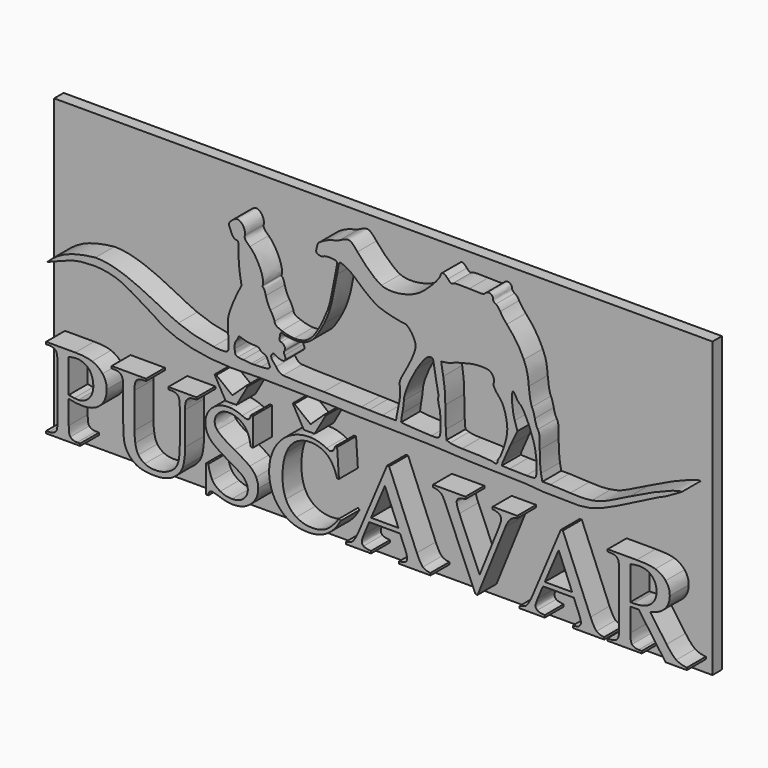
from build123d import *

# Parameters (mm, degrees)
F1_DEPTH = 2
F2_W     = 55.653892
F2_H     = 24.8238056814
F3_DEPTH = 1


# Not quite as in the source:
# - ends of sketch curves that miss each other by under 0.0002 mm in the source are joined


with BuildPart() as f1:
    # F0 (on Front) → F1 (new body)
    with BuildSketch(Plane.XZ):
        with BuildLine():
            add(Edge.make_bspline(
                [(-25.170871, -10.131624), (-25.170873, -10.560896), (-25.124563, -10.827515), (-25.031942, -10.931476)],
                knots=[0, 0, 0, 0, 1, 1, 1, 1], degree=3))
            Line((-25.170871, -10.131624), (-25.170871, -8.14457))
            add(Edge.make_bspline(
                [(-24.565539, -8.250211), (-24.754088, -8.226738), (-24.955865, -8.191524), (-25.170871, -8.14457)],
                knots=[0, 0, 0, 0, 1, 1, 1, 1], degree=3))
            add(Edge.make_bspline(
                [(-24.039596, -8.285425), (-24.201682, -8.285428), (-24.376996, -8.273689), (-24.565539, -8.250211)],
                knots=[0, 0, 0, 0, 1, 1, 1, 1], degree=3))
            add(Edge.make_bspline(
                [(-22.503939, -7.762251), (-22.86615, -8.111038), (-23.378035, -8.285428), (-24.039596, -8.285425)],
                knots=[0, 0, 0, 0, 1, 1, 1, 1], degree=3))
            add(Edge.make_bspline(
                [(-21.96063, -6.40401), (-21.960635, -6.960725), (-22.141738, -7.413473), (-22.503939, -7.762251)],
                knots=[0, 0, 0, 0, 1, 1, 1, 1], degree=3))
            add(Edge.make_bspline(
                [(-22.317874, -5.342571), (-22.079716, -5.641054), (-21.960635, -5.994868), (-21.96063, -6.40401)],
                knots=[0, 0, 0, 0, 1, 1, 1, 1], degree=3))
            add(Edge.make_bspline(
                [(-23.196101, -4.706211), (-22.848784, -4.83198), (-22.556042, -5.0441), (-22.317874, -5.342571)],
                knots=[0, 0, 0, 0, 1, 1, 1, 1], degree=3))
            add(Edge.make_bspline(
                [(-24.620119, -4.517567), (-24.018098, -4.517572), (-23.543426, -4.580454), (-23.196101, -4.706211)],
                knots=[0, 0, 0, 0, 1, 1, 1, 1], degree=3))
            Line((-24.620119, -4.517567), (-27.0861, -4.517567))
            Line((-27.0861, -4.517567), (-27.0861, -4.703696))
            Line((-27.0861, -4.703696), (-26.833052, -4.703696))
            add(Edge.make_bspline(
                [(-26.257491, -4.925038), (-26.386496, -4.777484), (-26.57835, -4.703702), (-26.833052, -4.703696)],
                knots=[0, 0, 0, 0, 1, 1, 1, 1], degree=3))
            add(Edge.make_bspline(
                [(-26.123524, -5.72489), (-26.123525, -5.295626), (-26.16818, -5.029008), (-26.257491, -4.925038)],
                knots=[0, 0, 0, 0, 1, 1, 1, 1], degree=3))
            Line((-26.123524, -5.72489), (-26.123524, -10.131624))
            add(Edge.make_bspline(
                [(-26.222758, -10.87111), (-26.156603, -10.767148), (-26.123525, -10.520652), (-26.123524, -10.131624)],
                knots=[0, 0, 0, 0, 1, 1, 1, 1], degree=3))
            add(Edge.make_bspline(
                [(-26.833052, -11.15282), (-26.548579, -11.15282), (-26.345149, -11.058916), (-26.222758, -10.87111)],
                knots=[0, 0, 0, 0, 1, 1, 1, 1], degree=3))
            Line((-26.833052, -11.15282), (-27.0861, -11.15282))
            Line((-27.0861, -11.15282), (-27.0861, -11.33895))
            Line((-27.0861, -11.33895), (-24.203333, -11.33895))
            Line((-24.203333, -11.33895), (-24.203333, -11.15282))
            Line((-24.203333, -11.15282), (-24.461343, -11.15282))
            add(Edge.make_bspline(
                [(-25.031942, -10.931476), (-24.906248, -11.079038), (-24.716048, -11.15282), (-24.461343, -11.15282)],
                knots=[0, 0, 0, 0, 1, 1, 1, 1], degree=3))
        make_face()
        with BuildLine():
            add(Edge.make_bspline(
                [(-25.170871, -7.857829), (-24.995558, -7.89137), (-24.840091, -7.916522), (-24.704468, -7.933288)],
                knots=[0, 0, 0, 0, 1, 1, 1, 1], degree=3))
            Line((-25.170871, -7.857829), (-25.170871, -5.020616))
            add(Edge.make_bspline(
                [(-24.520884, -4.925035), (-24.689585, -4.925041), (-24.906248, -4.956902), (-25.170871, -5.020616)],
                knots=[0, 0, 0, 0, 1, 1, 1, 1], degree=3))
            add(Edge.make_bspline(
                [(-23.776624, -5.11368), (-23.994943, -4.987922), (-24.24303, -4.925041), (-24.520884, -4.925035)],
                knots=[0, 0, 0, 0, 1, 1, 1, 1], degree=3))
            add(Edge.make_bspline(
                [(-23.270527, -5.682128), (-23.389612, -5.428931), (-23.558311, -5.239448), (-23.776624, -5.11368)],
                knots=[0, 0, 0, 0, 1, 1, 1, 1], degree=3))
            add(Edge.make_bspline(
                [(-23.091905, -6.504618), (-23.091909, -6.2095), (-23.15145, -5.935336), (-23.270527, -5.682128)],
                knots=[0, 0, 0, 0, 1, 1, 1, 1], degree=3))
            add(Edge.make_bspline(
                [(-23.466516, -7.553481), (-23.216779, -7.283515), (-23.091909, -6.933893), (-23.091905, -6.504618)],
                knots=[0, 0, 0, 0, 1, 1, 1, 1], degree=3))
            add(Edge.make_bspline(
                [(-24.357147, -7.958437), (-24.013136, -7.95844), (-23.71626, -7.823456), (-23.466516, -7.553481)],
                knots=[0, 0, 0, 0, 1, 1, 1, 1], degree=3))
            add(Edge.make_bspline(
                [(-24.704468, -7.933288), (-24.56885, -7.950054), (-24.453076, -7.958437), (-24.357147, -7.958437)],
                knots=[0, 0, 0, 0, 1, 1, 1, 1], degree=3))
        make_face(mode=Mode.SUBTRACT)
    extrude(amount=F1_DEPTH)



with BuildPart() as f1b:
    # F0 (on Front) → F1, piece 2 (new body)
    with BuildSketch(Plane.XZ):
        with BuildLine():
            add(Edge.make_bspline(
                [(-14.622226, -4.703696), (-14.886858, -4.703702), (-15.09029, -4.816049), (-15.23252, -5.040741)],
                knots=[0, 0, 0, 0, 1, 1, 1, 1], degree=3))
            Line((-14.622226, -4.703696), (-14.369178, -4.703696))
            Line((-14.369178, -4.703696), (-14.369178, -4.517567))
            Line((-14.369178, -4.517567), (-16.75081, -4.517567))
            Line((-16.75081, -4.517567), (-16.75081, -4.703696))
            Line((-16.75081, -4.703696), (-16.497762, -4.703696))
            add(Edge.make_bspline(
                [(-15.922201, -4.925038), (-16.051211, -4.777484), (-16.243065, -4.703702), (-16.497762, -4.703696)],
                knots=[0, 0, 0, 0, 1, 1, 1, 1], degree=3))
            add(Edge.make_bspline(
                [(-15.783272, -5.72489), (-15.783278, -5.298979), (-15.829587, -5.032364), (-15.922201, -4.925038)],
                knots=[0, 0, 0, 0, 1, 1, 1, 1], degree=3))
            Line((-15.783272, -5.72489), (-15.783272, -8.486644))
            add(Edge.make_bspline(
                [(-15.974299, -10.028498), (-15.846953, -9.724994), (-15.783278, -9.211041), (-15.783272, -8.486644)],
                knots=[0, 0, 0, 0, 1, 1, 1, 1], degree=3))
            add(Edge.make_bspline(
                [(-16.686307, -10.775531), (-16.338991, -10.581019), (-16.101656, -10.332007), (-15.974299, -10.028498)],
                knots=[0, 0, 0, 0, 1, 1, 1, 1], degree=3))
            add(Edge.make_bspline(
                [(-17.8672, -11.067302), (-17.427264, -11.067302), (-17.033633, -10.970044), (-16.686307, -10.775531)],
                knots=[0, 0, 0, 0, 1, 1, 1, 1], degree=3))
            add(Edge.make_bspline(
                [(-18.737984, -10.881172), (-18.501478, -11.005259), (-18.211217, -11.067302), (-17.8672, -11.067302)],
                knots=[0, 0, 0, 0, 1, 1, 1, 1], degree=3))
            add(Edge.make_bspline(
                [(-19.281294, -10.408302), (-19.155599, -10.599464), (-18.974496, -10.757086), (-18.737984, -10.881172)],
                knots=[0, 0, 0, 0, 1, 1, 1, 1], degree=3))
            add(Edge.make_bspline(
                [(-19.541785, -9.608452), (-19.493824, -9.950527), (-19.406993, -10.217145), (-19.281294, -10.408302)],
                knots=[0, 0, 0, 0, 1, 1, 1, 1], degree=3))
            add(Edge.make_bspline(
                [(-19.61373, -8.697926), (-19.613732, -8.962871), (-19.589751, -9.266378), (-19.541785, -9.608452)],
                knots=[0, 0, 0, 0, 1, 1, 1, 1], degree=3))
            Line((-19.61373, -8.697926), (-19.61373, -5.72489))
            add(Edge.make_bspline(
                [(-19.489687, -4.970312), (-19.572384, -5.091051), (-19.613732, -5.342577), (-19.61373, -5.72489)],
                knots=[0, 0, 0, 0, 1, 1, 1, 1], degree=3))
            add(Edge.make_bspline(
                [(-18.894279, -4.703696), (-19.172138, -4.703702), (-19.370607, -4.792574), (-19.489687, -4.970312)],
                knots=[0, 0, 0, 0, 1, 1, 1, 1], degree=3))
            Line((-18.894279, -4.703696), (-18.636269, -4.703696))
            Line((-18.636269, -4.703696), (-18.636269, -4.517567))
            Line((-18.636269, -4.517567), (-21.543844, -4.517567))
            Line((-21.543844, -4.517567), (-21.543844, -4.703696))
            Line((-21.543844, -4.703696), (-21.290796, -4.703696))
            add(Edge.make_bspline(
                [(-20.737563, -4.899886), (-20.851683, -4.769099), (-21.036094, -4.703702), (-21.290796, -4.703696)],
                knots=[0, 0, 0, 0, 1, 1, 1, 1], degree=3))
            add(Edge.make_bspline(
                [(-20.566383, -5.72489), (-20.566384, -5.305686), (-20.623444, -5.030684), (-20.737563, -4.899886)],
                knots=[0, 0, 0, 0, 1, 1, 1, 1], degree=3))
            Line((-20.566383, -5.72489), (-20.566383, -8.391066))
            add(Edge.make_bspline(
                [(-20.407607, -10.071257), (-20.513459, -9.772783), (-20.566384, -9.212717), (-20.566383, -8.391066)],
                knots=[0, 0, 0, 0, 1, 1, 1, 1], degree=3))
            add(Edge.make_bspline(
                [(-19.598845, -11.112576), (-19.979246, -10.854343), (-20.248833, -10.507236), (-20.407607, -10.071257)],
                knots=[0, 0, 0, 0, 1, 1, 1, 1], degree=3))
            add(Edge.make_bspline(
                [(-17.926741, -11.499925), (-18.66108, -11.499925), (-19.218448, -11.370808), (-19.598845, -11.112576)],
                knots=[0, 0, 0, 0, 1, 1, 1, 1], degree=3))
            add(Edge.make_bspline(
                [(-16.326582, -11.094969), (-16.718564, -11.36494), (-17.251949, -11.499925), (-17.926741, -11.499925)],
                knots=[0, 0, 0, 0, 1, 1, 1, 1], degree=3))
            add(Edge.make_bspline(
                [(-15.537666, -10.124079), (-15.671639, -10.501368), (-15.934611, -10.824997), (-16.326582, -11.094969)],
                knots=[0, 0, 0, 0, 1, 1, 1, 1], degree=3))
            add(Edge.make_bspline(
                [(-15.336716, -8.531919), (-15.336722, -9.216074), (-15.403706, -9.746793), (-15.537666, -10.124079)],
                knots=[0, 0, 0, 0, 1, 1, 1, 1], degree=3))
            Line((-15.336716, -8.531919), (-15.336716, -5.765135))
            add(Edge.make_bspline(
                [(-15.23252, -5.040741), (-15.30199, -5.144711), (-15.336722, -5.386175), (-15.336716, -5.765135)],
                knots=[0, 0, 0, 0, 1, 1, 1, 1], degree=3))
        make_face()
    extrude(amount=F1_DEPTH)


with BuildPart() as f1c:
    # F0 (on Front) → F1, piece 3 (new body)
    with BuildSketch(Plane.XZ):
        with BuildLine():
            add(Edge.make_bspline(
                [(-9.779574, -6.720932), (-9.839121, -6.268193), (-9.945798, -5.907672), (-10.099608, -5.639372)],
                knots=[0, 0, 0, 0, 1, 1, 1, 1], degree=3))
            Line((-9.779574, -6.720932), (-9.59599, -6.720932))
            Line((-9.59599, -6.720932), (-9.59599, -4.361619))
            Line((-9.59599, -4.361619), (-9.779574, -4.361619))
            add(Edge.make_bspline(
                [(-9.911059, -4.676027), (-9.856485, -4.624052), (-9.812656, -4.519249), (-9.779574, -4.361619)],
                knots=[0, 0, 0, 0, 1, 1, 1, 1], degree=3))
            add(Edge.make_bspline(
                [(-10.121935, -4.754001), (-10.035935, -4.754006), (-9.965645, -4.728027), (-9.911059, -4.676027)],
                knots=[0, 0, 0, 0, 1, 1, 1, 1], degree=3))
            add(Edge.make_bspline(
                [(-10.51391, -4.628237), (-10.328677, -4.712085), (-10.198019, -4.754006), (-10.121935, -4.754001)],
                knots=[0, 0, 0, 0, 1, 1, 1, 1], degree=3))
            add(Edge.make_bspline(
                [(-11.650148, -4.361619), (-11.292906, -4.361628), (-10.914161, -4.450499), (-10.51391, -4.628237)],
                knots=[0, 0, 0, 0, 1, 1, 1, 1], degree=3))
            add(Edge.make_bspline(
                [(-13.064241, -4.892341), (-12.693768, -4.538533), (-12.222402, -4.361628), (-11.650148, -4.361619)],
                knots=[0, 0, 0, 0, 1, 1, 1, 1], degree=3))
            add(Edge.make_bspline(
                [(-13.619956, -6.157516), (-13.619956, -5.667883), (-13.434718, -5.24616), (-13.064241, -4.892341)],
                knots=[0, 0, 0, 0, 1, 1, 1, 1], degree=3))
            add(Edge.make_bspline(
                [(-13.431411, -6.932214), (-13.557108, -6.697462), (-13.619956, -6.43923), (-13.619956, -6.157516)],
                knots=[0, 0, 0, 0, 1, 1, 1, 1], degree=3))
            add(Edge.make_bspline(
                [(-12.878176, -7.576121), (-13.121302, -7.381611), (-13.305713, -7.166977), (-13.431411, -6.932214)],
                knots=[0, 0, 0, 0, 1, 1, 1, 1], degree=3))
            add(Edge.make_bspline(
                [(-11.650148, -8.358367), (-12.225712, -8.031387), (-12.635053, -7.77064), (-12.878176, -7.576121)],
                knots=[0, 0, 0, 0, 1, 1, 1, 1], degree=3))
            add(Edge.make_bspline(
                [(-10.593298, -8.999759), (-10.722308, -8.899151), (-11.074591, -8.685354), (-11.650148, -8.358367)],
                knots=[0, 0, 0, 0, 1, 1, 1, 1], degree=3))
            add(Edge.make_bspline(
                [(-10.169071, -9.477656), (-10.260041, -9.306622), (-10.401448, -9.147321), (-10.593298, -8.999759)],
                knots=[0, 0, 0, 0, 1, 1, 1, 1], degree=3))
            add(Edge.make_bspline(
                [(-10.032622, -9.985738), (-10.032628, -9.818057), (-10.07811, -9.648697), (-10.169071, -9.477656)],
                knots=[0, 0, 0, 0, 1, 1, 1, 1], degree=3))
            add(Edge.make_bspline(
                [(-10.39235, -10.770501), (-10.152537, -10.549157), (-10.032628, -10.287571), (-10.032622, -9.985738)],
                knots=[0, 0, 0, 0, 1, 1, 1, 1], degree=3))
            add(Edge.make_bspline(
                [(-11.372292, -11.102513), (-10.958816, -11.102516), (-10.632168, -10.991843), (-10.39235, -10.770501)],
                knots=[0, 0, 0, 0, 1, 1, 1, 1], degree=3))
            add(Edge.make_bspline(
                [(-12.357194, -10.86105), (-12.057841, -11.022027), (-11.729539, -11.102516), (-11.372292, -11.102513)],
                knots=[0, 0, 0, 0, 1, 1, 1, 1], degree=3))
            add(Edge.make_bspline(
                [(-13.024547, -10.254872), (-12.879006, -10.498015), (-12.656554, -10.700075), (-12.357194, -10.86105)],
                knots=[0, 0, 0, 0, 1, 1, 1, 1], degree=3))
            add(Edge.make_bspline(
                [(-13.371869, -9.155704), (-13.285866, -9.645343), (-13.170094, -10.011732), (-13.024547, -10.254872)],
                knots=[0, 0, 0, 0, 1, 1, 1, 1], degree=3))
            Line((-13.371869, -9.155704), (-13.555454, -9.155704))
            Line((-13.555454, -9.155704), (-13.555454, -11.494895))
            Line((-13.555454, -11.494895), (-13.371869, -11.494895))
            add(Edge.make_bspline(
                [(-13.265192, -11.183002), (-13.313155, -11.233309), (-13.348715, -11.337273), (-13.371869, -11.494895)],
                knots=[0, 0, 0, 0, 1, 1, 1, 1], degree=3))
            add(Edge.make_bspline(
                [(-13.069202, -11.107546), (-13.151901, -11.107546), (-13.21723, -11.132695), (-13.265192, -11.183002)],
                knots=[0, 0, 0, 0, 1, 1, 1, 1], degree=3))
            add(Edge.make_bspline(
                [(-12.45643, -11.266006), (-12.778944, -11.160365), (-12.983202, -11.107546), (-13.069202, -11.107546)],
                knots=[0, 0, 0, 0, 1, 1, 1, 1], degree=3))
            add(Edge.make_bspline(
                [(-11.818846, -11.449621), (-11.921392, -11.432855), (-12.133919, -11.371647), (-12.45643, -11.266006)],
                knots=[0, 0, 0, 0, 1, 1, 1, 1], degree=3))
            add(Edge.make_bspline(
                [(-11.268095, -11.494895), (-11.463258, -11.494895), (-11.646843, -11.479805), (-11.818846, -11.449621)],
                knots=[0, 0, 0, 0, 1, 1, 1, 1], degree=3))
            add(Edge.make_bspline(
                [(-9.742361, -10.933991), (-10.137651, -11.307927), (-10.646227, -11.494895), (-11.268095, -11.494895)],
                knots=[0, 0, 0, 0, 1, 1, 1, 1], degree=3))
            add(Edge.make_bspline(
                [(-9.149435, -9.59839), (-9.149441, -10.114858), (-9.347082, -10.560058), (-9.742361, -10.933991)],
                knots=[0, 0, 0, 0, 1, 1, 1, 1], degree=3))
            add(Edge.make_bspline(
                [(-9.3355, -8.818659), (-9.211462, -9.066835), (-9.149441, -9.326744), (-9.149435, -9.59839)],
                knots=[0, 0, 0, 0, 1, 1, 1, 1], degree=3))
            add(Edge.make_bspline(
                [(-9.866404, -8.172237), (-9.636516, -8.355016), (-9.459546, -8.570489), (-9.3355, -8.818659)],
                knots=[0, 0, 0, 0, 1, 1, 1, 1], degree=3))
            add(Edge.make_bspline(
                [(-11.153974, -7.384962), (-10.525491, -7.727039), (-10.096303, -7.989466), (-9.866404, -8.172237)],
                knots=[0, 0, 0, 0, 1, 1, 1, 1], degree=3))
            add(Edge.make_bspline(
                [(-12.617687, -6.378858), (-12.412601, -6.630389), (-11.924699, -6.965757), (-11.153974, -7.384962)],
                knots=[0, 0, 0, 0, 1, 1, 1, 1], degree=3))
            add(Edge.make_bspline(
                [(-12.831041, -5.810409), (-12.831041, -6.018343), (-12.759924, -6.207826), (-12.617687, -6.378858)],
                knots=[0, 0, 0, 0, 1, 1, 1, 1], degree=3))
            add(Edge.make_bspline(
                [(-12.493643, -5.0835), (-12.718576, -5.296464), (-12.831041, -5.538766), (-12.831041, -5.810409)],
                knots=[0, 0, 0, 0, 1, 1, 1, 1], degree=3))
            add(Edge.make_bspline(
                [(-11.640225, -4.764063), (-11.98424, -4.764069), (-12.268714, -4.870548), (-12.493643, -5.0835)],
                knots=[0, 0, 0, 0, 1, 1, 1, 1], degree=3))
            add(Edge.make_bspline(
                [(-10.757036, -5.000497), (-11.041512, -4.842881), (-11.335908, -4.764069), (-11.640225, -4.764063)],
                knots=[0, 0, 0, 0, 1, 1, 1, 1], degree=3))
            add(Edge.make_bspline(
                [(-10.099608, -5.639372), (-10.253423, -5.371082), (-10.472568, -5.158124), (-10.757036, -5.000497)],
                knots=[0, 0, 0, 0, 1, 1, 1, 1], degree=3))
        make_face()
    extrude(amount=F1_DEPTH)


with BuildPart() as f1d:
    # F0 (on Front) → F1, piece 4 (new body)
    with BuildSketch(Plane.XZ):
        Polygon((-11.903195, -3.984333), (-10.990236, -3.984333), (-10.052469, -2.319231), (-10.201321, -2.319231), (-11.337559, -3.385699), (-12.692111, -2.319231), (-12.845927, -2.319231), align=None)
    extrude(amount=F1_DEPTH)


with BuildPart() as f1e:
    # F0 (on Front) → F1, piece 5 (new body)
    with BuildSketch(Plane.XZ):
        with BuildLine():
            add(Edge.make_bspline(
                [(-2.480866, -6.680691), (-2.685956, -5.986482), (-2.978698, -5.486786), (-3.359094, -5.181594)],
                knots=[0, 0, 0, 0, 1, 1, 1, 1], degree=3))
            Line((-2.480866, -6.680691), (-2.327053, -6.680691))
            Line((-2.327053, -6.680691), (-2.480866, -4.361619))
            Line((-2.480866, -4.361619), (-2.654528, -4.361619))
            add(Edge.make_bspline(
                [(-2.838113, -4.738908), (-2.752112, -4.648365), (-2.69092, -4.522605), (-2.654528, -4.361619)],
                knots=[0, 0, 0, 0, 1, 1, 1, 1], degree=3))
            add(Edge.make_bspline(
                [(-3.071313, -4.834489), (-2.982006, -4.834495), (-2.904274, -4.802636), (-2.838113, -4.738908)],
                knots=[0, 0, 0, 0, 1, 1, 1, 1], degree=3))
            add(Edge.make_bspline(
                [(-3.369016, -4.723819), (-3.230093, -4.797604), (-3.13086, -4.834495), (-3.071313, -4.834489)],
                knots=[0, 0, 0, 0, 1, 1, 1, 1], degree=3))
            add(Edge.make_bspline(
                [(-4.807918, -4.361619), (-4.321672, -4.361628), (-3.842041, -4.482361), (-3.369016, -4.723819)],
                knots=[0, 0, 0, 0, 1, 1, 1, 1], degree=3))
            add(Edge.make_bspline(
                [(-6.537085, -4.831974), (-6.009488, -4.518411), (-5.433102, -4.361628), (-4.807918, -4.361619)],
                knots=[0, 0, 0, 0, 1, 1, 1, 1], degree=3))
            add(Edge.make_bspline(
                [(-7.779996, -6.157516), (-7.478986, -5.587397), (-7.064681, -5.145549), (-6.537085, -4.831974)],
                knots=[0, 0, 0, 0, 1, 1, 1, 1], degree=3))
            add(Edge.make_bspline(
                [(-8.231515, -8.033899), (-8.231515, -7.353106), (-8.08101, -6.727644), (-7.779996, -6.157516)],
                knots=[0, 0, 0, 0, 1, 1, 1, 1], degree=3))
            add(Edge.make_bspline(
                [(-7.546796, -10.237265), (-8.003275, -9.613482), (-8.231515, -8.879029), (-8.231515, -8.033899)],
                knots=[0, 0, 0, 0, 1, 1, 1, 1], degree=3))
            add(Edge.make_bspline(
                [(-4.95677, -11.494895), (-6.07151, -11.494895), (-6.93485, -11.075685), (-7.546796, -10.237265)],
                knots=[0, 0, 0, 0, 1, 1, 1, 1], degree=3))
            add(Edge.make_bspline(
                [(-3.35413, -11.072332), (-3.804001, -11.35404), (-4.338212, -11.494895), (-4.95677, -11.494895)],
                knots=[0, 0, 0, 0, 1, 1, 1, 1], degree=3))
            add(Edge.make_bspline(
                [(-2.17324, -9.739245), (-2.510643, -10.346261), (-2.904274, -10.790624), (-3.35413, -11.072332)],
                knots=[0, 0, 0, 0, 1, 1, 1, 1], degree=3))
            Line((-2.17324, -9.739245), (-2.327053, -9.638634))
            add(Edge.make_bspline(
                [(-3.428558, -10.767986), (-3.094473, -10.578504), (-2.727304, -10.202053), (-2.327053, -9.638634)],
                knots=[0, 0, 0, 0, 1, 1, 1, 1], degree=3))
            add(Edge.make_bspline(
                [(-4.584642, -11.052209), (-4.148013, -11.052209), (-3.762653, -10.957469), (-3.428558, -10.767986)],
                knots=[0, 0, 0, 0, 1, 1, 1, 1], degree=3))
            add(Edge.make_bspline(
                [(-5.92679, -10.690013), (-5.534815, -10.931476), (-5.087434, -11.052209), (-4.584642, -11.052209)],
                knots=[0, 0, 0, 0, 1, 1, 1, 1], degree=3))
            add(Edge.make_bspline(
                [(-6.807499, -9.648694), (-6.612339, -10.101442), (-6.31877, -10.448549), (-5.92679, -10.690013)],
                knots=[0, 0, 0, 0, 1, 1, 1, 1], degree=3))
            add(Edge.make_bspline(
                [(-7.100241, -8.043959), (-7.100241, -8.661038), (-7.002662, -9.195951), (-6.807499, -9.648694)],
                knots=[0, 0, 0, 0, 1, 1, 1, 1], degree=3))
            add(Edge.make_bspline(
                [(-6.790132, -6.167576), (-6.996871, -6.670634), (-7.100241, -7.296093), (-7.100241, -8.043959)],
                knots=[0, 0, 0, 0, 1, 1, 1, 1], degree=3))
            add(Edge.make_bspline(
                [(-5.939195, -5.068408), (-6.29975, -5.298141), (-6.583393, -5.664529), (-6.790132, -6.167576)],
                knots=[0, 0, 0, 0, 1, 1, 1, 1], degree=3))
            add(Edge.make_bspline(
                [(-4.728533, -4.723819), (-5.17509, -4.723824), (-5.578643, -4.838687), (-5.939195, -5.068408)],
                knots=[0, 0, 0, 0, 1, 1, 1, 1], degree=3))
            add(Edge.make_bspline(
                [(-3.359094, -5.181594), (-3.739499, -4.876416), (-4.195975, -4.723824), (-4.728533, -4.723819)],
                knots=[0, 0, 0, 0, 1, 1, 1, 1], degree=3))
        make_face()
    extrude(amount=F1_DEPTH)


with BuildPart() as f1f:
    # F0 (on Front) → F1, piece 6 (new body)
    with BuildSketch(Plane.XZ):
        Polygon((-5.29417, -3.984333), (-4.381211, -3.984333), (-3.443444, -2.319231), (-3.592295, -2.319231), (-4.728533, -3.385699), (-6.083086, -2.319231), (-6.236898, -2.319231), align=None)
    extrude(amount=F1_DEPTH)


with BuildPart() as f1g:
    # F0 (on Front) → F1, piece 7 (new body)
    with BuildSketch(Plane.XZ):
        with BuildLine():
            add(Edge.make_bspline(
                [(-0.223279, -10.131624), (-0.335746, -10.396565), (-0.391977, -10.594434), (-0.391977, -10.725227)],
                knots=[0, 0, 0, 0, 1, 1, 1, 1], degree=3))
            Line((-0.223279, -10.131624), (0.233201, -9.055093))
            Line((0.233201, -9.055093), (2.838112, -9.055093))
            Line((2.838112, -9.055093), (3.244973, -10.036045))
            add(Edge.make_bspline(
                [(3.443444, -10.735287), (3.443438, -10.587725), (3.377282, -10.354644), (3.244973, -10.036045)],
                knots=[0, 0, 0, 0, 1, 1, 1, 1], degree=3))
            add(Edge.make_bspline(
                [(3.302034, -11.016995), (3.396302, -10.939862), (3.443438, -10.845958), (3.443444, -10.735287)],
                knots=[0, 0, 0, 0, 1, 1, 1, 1], degree=3))
            add(Edge.make_bspline(
                [(2.758724, -11.15282), (3.026652, -11.139407), (3.207757, -11.09413), (3.302034, -11.016995)],
                knots=[0, 0, 0, 0, 1, 1, 1, 1], degree=3))
            Line((2.758724, -11.15282), (2.758724, -11.33895))
            Line((2.758724, -11.33895), (5.413249, -11.33895))
            Line((5.413249, -11.33895), (5.413249, -11.15282))
            add(Edge.make_bspline(
                [(4.770707, -10.923931), (4.924514, -11.059754), (5.138695, -11.136051), (5.413249, -11.15282)],
                knots=[0, 0, 0, 0, 1, 1, 1, 1], degree=3))
            add(Edge.make_bspline(
                [(4.257167, -10.036045), (4.445707, -10.492147), (4.616886, -10.788109), (4.770707, -10.923931)],
                knots=[0, 0, 0, 0, 1, 1, 1, 1], degree=3))
            Line((4.257167, -10.036045), (1.915228, -4.361619))
            Line((1.915228, -4.361619), (1.741569, -4.361619))
            Line((1.741569, -4.361619), (-0.625178, -9.975679))
            add(Edge.make_bspline(
                [(-1.185854, -10.956628), (-1.017155, -10.795653), (-0.830264, -10.468671), (-0.625178, -9.975679)],
                knots=[0, 0, 0, 0, 1, 1, 1, 1], degree=3))
            add(Edge.make_bspline(
                [(-1.731644, -11.15282), (-1.450481, -11.102516), (-1.26855, -11.037117), (-1.185854, -10.956628)],
                knots=[0, 0, 0, 0, 1, 1, 1, 1], degree=3))
            Line((-1.731644, -11.15282), (-1.731644, -11.33895))
            Line((-1.731644, -11.33895), (0.387016, -11.33895))
            Line((0.387016, -11.33895), (0.387016, -11.15282))
            add(Edge.make_bspline(
                [(-0.245606, -10.99939), (-0.148028, -11.0782), (0.062846, -11.129345), (0.387016, -11.15282)],
                knots=[0, 0, 0, 0, 1, 1, 1, 1], degree=3))
            add(Edge.make_bspline(
                [(-0.391977, -10.725227), (-0.391977, -10.829191), (-0.343188, -10.920578), (-0.245606, -10.99939)],
                knots=[0, 0, 0, 0, 1, 1, 1, 1], degree=3))
        make_face()
        Polygon((1.557984, -5.926112), (2.699183, -8.682837), (0.387016, -8.682837), align=None, mode=Mode.SUBTRACT)
    extrude(amount=F1_DEPTH)


with BuildPart() as f1h:
    # F0 (on Front) → F1, piece 8 (new body)
    with BuildSketch(Plane.XZ):
        with BuildLine():
            add(Edge.make_bspline(
                [(12.746691, -4.703696), (12.508521, -4.7473), (12.328246, -4.824435), (12.205862, -4.9351)],
                knots=[0, 0, 0, 0, 1, 1, 1, 1], degree=3))
            Line((12.746691, -4.703696), (12.746691, -4.517567))
            Line((12.746691, -4.517567), (10.672686, -4.517567))
            Line((10.672686, -4.517567), (10.672686, -4.703696))
            add(Edge.make_bspline(
                [(10.757035, -4.718786), (10.740499, -4.715433), (10.712375, -4.710403), (10.672686, -4.703696)],
                knots=[0, 0, 0, 0, 1, 1, 1, 1], degree=3))
            add(Edge.make_bspline(
                [(11.243287, -4.907431), (11.147353, -4.818564), (10.98527, -4.755683), (10.757035, -4.718786)],
                knots=[0, 0, 0, 0, 1, 1, 1, 1], degree=3))
            add(Edge.make_bspline(
                [(11.387177, -5.186626), (11.387172, -5.089374), (11.339206, -4.996311), (11.243287, -4.907431)],
                knots=[0, 0, 0, 0, 1, 1, 1, 1], degree=3))
            add(Edge.make_bspline(
                [(11.153974, -5.996539), (11.309437, -5.607519), (11.387172, -5.337547), (11.387177, -5.186626)],
                knots=[0, 0, 0, 0, 1, 1, 1, 1], degree=3))
            Line((11.153974, -5.996539), (9.56622, -9.945497))
            Line((9.56622, -9.945497), (7.854423, -5.946234))
            add(Edge.make_bspline(
                [(7.626184, -5.161472), (7.626181, -5.329164), (7.702262, -5.59075), (7.854423, -5.946234)],
                knots=[0, 0, 0, 0, 1, 1, 1, 1], degree=3))
            add(Edge.make_bspline(
                [(7.76511, -4.864671), (7.67249, -4.941812), (7.626181, -5.040747), (7.626184, -5.161472)],
                knots=[0, 0, 0, 0, 1, 1, 1, 1], degree=3))
            add(Edge.make_bspline(
                [(8.370444, -4.703696), (8.059506, -4.733884), (7.857728, -4.787544), (7.76511, -4.864671)],
                knots=[0, 0, 0, 0, 1, 1, 1, 1], degree=3))
            Line((8.370444, -4.703696), (8.370444, -4.517567))
            Line((8.370444, -4.517567), (5.621642, -4.517567))
            Line((5.621642, -4.517567), (5.621642, -4.703696))
            add(Edge.make_bspline(
                [(6.110374, -4.816882), (5.989638, -4.758201), (5.826727, -4.720471), (5.621642, -4.703696)],
                knots=[0, 0, 0, 0, 1, 1, 1, 1], degree=3))
            add(Edge.make_bspline(
                [(6.415519, -5.060863), (6.332823, -4.956905), (6.231107, -4.875578), (6.110374, -4.816882)],
                knots=[0, 0, 0, 0, 1, 1, 1, 1], degree=3))
            add(Edge.make_bspline(
                [(6.688417, -5.61422), (6.559409, -5.312395), (6.468445, -5.127942), (6.415519, -5.060863)],
                knots=[0, 0, 0, 0, 1, 1, 1, 1], degree=3))
            Line((6.688417, -5.61422), (9.208976, -11.494895))
            Line((9.208976, -11.494895), (9.392561, -11.494895))
            Line((9.392561, -11.494895), (11.739461, -5.689679))
            add(Edge.make_bspline(
                [(12.205862, -4.9351), (12.030541, -5.099437), (11.875074, -5.350963), (11.739461, -5.689679)],
                knots=[0, 0, 0, 0, 1, 1, 1, 1], degree=3))
        make_face()
    extrude(amount=F1_DEPTH)


with BuildPart() as f1i:
    # F0 (on Front) → F1, piece 9 (new body)
    with BuildSketch(Plane.XZ):
        with BuildLine():
            add(Edge.make_bspline(
                [(14.463452, -10.131624), (14.350984, -10.396565), (14.294753, -10.594434), (14.294753, -10.725227)],
                knots=[0, 0, 0, 0, 1, 1, 1, 1], degree=3))
            Line((14.463452, -10.131624), (14.919931, -9.055093))
            Line((14.919931, -9.055093), (17.524843, -9.055093))
            Line((17.524843, -9.055093), (17.931704, -10.036045))
            add(Edge.make_bspline(
                [(18.130174, -10.735287), (18.130169, -10.587725), (18.064013, -10.354644), (17.931704, -10.036045)],
                knots=[0, 0, 0, 0, 1, 1, 1, 1], degree=3))
            add(Edge.make_bspline(
                [(17.988764, -11.016995), (18.083033, -10.939862), (18.130169, -10.845958), (18.130174, -10.735287)],
                knots=[0, 0, 0, 0, 1, 1, 1, 1], degree=3))
            add(Edge.make_bspline(
                [(17.445455, -11.15282), (17.713383, -11.139407), (17.894487, -11.09413), (17.988764, -11.016995)],
                knots=[0, 0, 0, 0, 1, 1, 1, 1], degree=3))
            Line((17.445455, -11.15282), (17.445455, -11.33895))
            Line((17.445455, -11.33895), (20.099983, -11.33895))
            Line((20.099983, -11.33895), (20.099983, -11.15282))
            add(Edge.make_bspline(
                [(19.457438, -10.923931), (19.611245, -11.059754), (19.825426, -11.136051), (20.099983, -11.15282)],
                knots=[0, 0, 0, 0, 1, 1, 1, 1], degree=3))
            add(Edge.make_bspline(
                [(18.943898, -10.036045), (19.132438, -10.492147), (19.303617, -10.788109), (19.457438, -10.923931)],
                knots=[0, 0, 0, 0, 1, 1, 1, 1], degree=3))
            Line((18.943898, -10.036045), (16.601959, -4.361619))
            Line((16.601959, -4.361619), (16.428299, -4.361619))
            Line((16.428299, -4.361619), (14.061552, -9.975679))
            add(Edge.make_bspline(
                [(13.500877, -10.956628), (13.669575, -10.795653), (13.856467, -10.468671), (14.061552, -9.975679)],
                knots=[0, 0, 0, 0, 1, 1, 1, 1], degree=3))
            add(Edge.make_bspline(
                [(12.955087, -11.15282), (13.23625, -11.102516), (13.418181, -11.037117), (13.500877, -10.956628)],
                knots=[0, 0, 0, 0, 1, 1, 1, 1], degree=3))
            Line((12.955087, -11.15282), (12.955087, -11.33895))
            Line((12.955087, -11.33895), (15.073747, -11.33895))
            Line((15.073747, -11.33895), (15.073747, -11.15282))
            add(Edge.make_bspline(
                [(14.441124, -10.99939), (14.538703, -11.0782), (14.749576, -11.129345), (15.073747, -11.15282)],
                knots=[0, 0, 0, 0, 1, 1, 1, 1], degree=3))
            add(Edge.make_bspline(
                [(14.294753, -10.725227), (14.294753, -10.829191), (14.343543, -10.920578), (14.441124, -10.99939)],
                knots=[0, 0, 0, 0, 1, 1, 1, 1], degree=3))
        make_face()
        Polygon((16.244715, -5.926112), (17.385914, -8.682837), (15.073747, -8.682837), align=None, mode=Mode.SUBTRACT)
    extrude(amount=F1_DEPTH)


with BuildPart() as f1j:
    # F0 (on Front) → F1, piece 10 (new body)
    with BuildSketch(Plane.XZ):
        with BuildLine():
            add(Edge.make_bspline(
                [(23.012517, -8.1496), (22.843815, -8.156306), (22.70654, -8.159659), (22.600692, -8.159659)],
                knots=[0, 0, 0, 0, 1, 1, 1, 1], degree=3))
            Line((23.012517, -8.1496), (25.289951, -11.33895))
            Line((25.289951, -11.33895), (27.0861, -11.33895))
            Line((27.0861, -11.33895), (27.0861, -11.152764))
            add(Edge.make_bspline(
                [(26.192988, -10.871053), (26.421222, -11.018617), (26.718925, -11.112519), (27.0861, -11.152764)],
                knots=[0, 0, 0, 0, 1, 1, 1, 1], degree=3))
            add(Edge.make_bspline(
                [(25.3743, -9.975622), (25.691847, -10.425017), (25.964742, -10.723494), (26.192988, -10.871053)],
                knots=[0, 0, 0, 0, 1, 1, 1, 1], degree=3))
            Line((25.3743, -9.975622), (23.985017, -8.01875))
            add(Edge.make_bspline(
                [(25.237854, -7.364783), (24.968261, -7.673325), (24.550648, -7.891313), (23.985017, -8.01875)],
                knots=[0, 0, 0, 0, 1, 1, 1, 1], degree=3))
            add(Edge.make_bspline(
                [(25.642234, -6.27316), (25.642228, -6.692376), (25.507436, -7.056249), (25.237854, -7.364783)],
                knots=[0, 0, 0, 0, 1, 1, 1, 1], degree=3))
            add(Edge.make_bspline(
                [(25.28747, -5.259511), (25.523976, -5.542904), (25.642228, -5.880787), (25.642234, -6.27316)],
                knots=[0, 0, 0, 0, 1, 1, 1, 1], degree=3))
            add(Edge.make_bspline(
                [(24.42413, -4.67597), (24.763175, -4.781619), (25.050956, -4.976132), (25.28747, -5.259511)],
                knots=[0, 0, 0, 0, 1, 1, 1, 1], degree=3))
            add(Edge.make_bspline(
                [(22.843818, -4.51751), (23.558304, -4.517516), (24.085074, -4.570337), (24.42413, -4.67597)],
                knots=[0, 0, 0, 0, 1, 1, 1, 1], degree=3))
            Line((22.843818, -4.51751), (20.392722, -4.51751))
            Line((20.392722, -4.51751), (20.392722, -4.70364))
            Line((20.392722, -4.70364), (20.64577, -4.70364))
            add(Edge.make_bspline(
                [(21.221332, -4.924981), (21.092324, -4.777428), (20.900471, -4.703645), (20.64577, -4.70364)],
                knots=[0, 0, 0, 0, 1, 1, 1, 1], degree=3))
            add(Edge.make_bspline(
                [(21.360258, -5.724833), (21.360258, -5.295569), (21.313949, -5.028951), (21.221332, -4.924981)],
                knots=[0, 0, 0, 0, 1, 1, 1, 1], degree=3))
            Line((21.360258, -5.724833), (21.360258, -10.131567))
            add(Edge.make_bspline(
                [(21.256062, -10.871053), (21.325525, -10.767091), (21.360258, -10.520595), (21.360258, -10.131567)],
                knots=[0, 0, 0, 0, 1, 1, 1, 1], degree=3))
            add(Edge.make_bspline(
                [(20.64577, -11.152764), (20.930241, -11.152764), (21.133672, -11.058859), (21.256062, -10.871053)],
                knots=[0, 0, 0, 0, 1, 1, 1, 1], degree=3))
            Line((20.64577, -11.152764), (20.392722, -11.152764))
            Line((20.392722, -11.152764), (20.392722, -11.338893))
            Line((20.392722, -11.338893), (23.275487, -11.338893))
            Line((23.275487, -11.338893), (23.275487, -11.152764))
            Line((23.275487, -11.152764), (23.012517, -11.152764))
            add(Edge.make_bspline(
                [(22.446877, -10.931419), (22.572574, -11.078981), (22.76112, -11.152764), (23.012517, -11.152764)],
                knots=[0, 0, 0, 0, 1, 1, 1, 1], degree=3))
            add(Edge.make_bspline(
                [(22.30795, -10.131567), (22.307948, -10.560839), (22.354257, -10.827458), (22.446877, -10.931419)],
                knots=[0, 0, 0, 0, 1, 1, 1, 1], degree=3))
            Line((22.30795, -10.131567), (22.30795, -8.149543))
            add(Edge.make_bspline(
                [(22.461763, -8.157102), (22.412144, -8.155397), (22.360874, -8.152925), (22.30795, -8.149543)],
                knots=[0, 0, 0, 0, 1, 1, 1, 1], degree=3))
            add(Edge.make_bspline(
                [(22.600692, -8.159659), (22.557688, -8.159662), (22.511379, -8.158807), (22.461763, -8.157102)],
                knots=[0, 0, 0, 0, 1, 1, 1, 1], degree=3))
        make_face()
        with BuildLine():
            add(Edge.make_bspline(
                [(22.30795, -7.832677), (22.370796, -7.83268), (22.425376, -7.83353), (22.471688, -7.835235)],
                knots=[0, 0, 0, 0, 1, 1, 1, 1], degree=3))
            Line((22.30795, -7.832677), (22.30795, -4.995552))
            add(Edge.make_bspline(
                [(23.086941, -4.899971), (22.895085, -4.899977), (22.635423, -4.931838), (22.30795, -4.995552)],
                knots=[0, 0, 0, 0, 1, 1, 1, 1], degree=3))
            add(Edge.make_bspline(
                [(24.131388, -5.299897), (23.868412, -5.033287), (23.520263, -4.899977), (23.086941, -4.899971)],
                knots=[0, 0, 0, 0, 1, 1, 1, 1], degree=3))
            add(Edge.make_bspline(
                [(24.525846, -6.338698), (24.52584, -5.912787), (24.394355, -5.566521), (24.131388, -5.299897)],
                knots=[0, 0, 0, 0, 1, 1, 1, 1], degree=3))
            add(Edge.make_bspline(
                [(24.037114, -7.415229), (24.36293, -7.133527), (24.52584, -6.774683), (24.525846, -6.338698)],
                knots=[0, 0, 0, 0, 1, 1, 1, 1], degree=3))
            add(Edge.make_bspline(
                [(22.585806, -7.837792), (23.227521, -7.837798), (23.71129, -7.696943), (24.037114, -7.415229)],
                knots=[0, 0, 0, 0, 1, 1, 1, 1], degree=3))
            add(Edge.make_bspline(
                [(22.471688, -7.835235), (22.517994, -7.83694), (22.556034, -7.837792), (22.585806, -7.837792)],
                knots=[0, 0, 0, 0, 1, 1, 1, 1], degree=3))
        make_face(mode=Mode.SUBTRACT)
    extrude(amount=F1_DEPTH)


with BuildPart() as f1k:
    # F0 (on Front) → F1, piece 11 (new body)
    with BuildSketch(Plane.XZ):
        with BuildLine():
            add(Edge.make_bspline(
                [(14.899742, -2.01623), (14.315567, -1.917706), (13.141794, -1.861118), (11.129629, -1.83447)],
                knots=[0, 0, 0, 0, 1, 1, 1, 1], degree=3))
            add(Edge.make_bspline(
                [(17.925147, -2.055885), (17.114303, -2.060683), (15.465705, -2.05295), (14.899742, -2.01623)],
                knots=[0, 0, 0, 0, 1, 1, 1, 1], degree=3))
            add(Edge.make_bspline(
                [(21.214684, -1.01897), (18.988603, -2.129127), (18.695713, -1.927172), (17.925147, -2.055885)],
                knots=[0, 0, 0, 0, 1, 1, 1, 1], degree=3))
            add(Edge.make_bspline(
                [(24.843422, 0.821794), (24.0324, 0.446125), (23.120621, -0.068468), (21.214684, -1.01897)],
                knots=[0, 0, 0, 0, 1, 1, 1, 1], degree=3))
            add(Edge.make_bspline(
                [(26.64895, 1.778186), (25.573248, 1.153286), (25.163936, 0.91725), (24.843422, 0.821794)],
                knots=[0, 0, 0, 0, 1, 1, 1, 1], degree=3))
            add(Edge.make_bspline(
                [(22.260445, 0.01807), (24.459105, 1.134149), (26.329982, 1.88451), (26.64895, 1.778186)],
                knots=[0, 0, 0, 0, 1, 1, 1, 1], degree=3))
            add(Edge.make_bspline(
                [(19.075084, -1.308662), (19.829797, -1.192646), (20.08362, -1.086926), (22.260445, 0.01807)],
                knots=[0, 0, 0, 0, 1, 1, 1, 1], degree=3))
            add(Edge.make_bspline(
                [(17.237152, -1.361023), (17.953776, -1.412909), (18.497725, -1.397413), (19.075084, -1.308662)],
                knots=[0, 0, 0, 0, 1, 1, 1, 1], degree=3))
            add(Edge.make_bspline(
                [(15.54574, -1.286872), (15.916188, -1.287134), (16.677324, -1.32049), (17.237152, -1.361023)],
                knots=[0, 0, 0, 0, 1, 1, 1, 1], degree=3))
            Line((15.54574, -1.286872), (14.8722, -1.286307))
            Line((14.8722, -1.286307), (14.753269, -0.709789))
            add(Edge.make_bspline(
                [(14.646597, 1.023368), (14.639852, 0.387217), (14.687858, -0.392704), (14.753269, -0.709789)],
                knots=[0, 0, 0, 0, 1, 1, 1, 1], degree=3))
            add(Edge.make_bspline(
                [(14.475681, 2.481218), (14.632946, 2.222612), (14.657121, 2.016407), (14.646597, 1.023368)],
                knots=[0, 0, 0, 0, 1, 1, 1, 1], degree=3))
            add(Edge.make_bspline(
                [(14.230288, 3.209637), (14.264508, 2.97467), (14.374933, 2.646883), (14.475681, 2.481218)],
                knots=[0, 0, 0, 0, 1, 1, 1, 1], degree=3))
            add(Edge.make_bspline(
                [(13.992815, 3.98485), (14.089208, 3.793447), (14.196072, 3.444601), (14.230288, 3.209637)],
                knots=[0, 0, 0, 0, 1, 1, 1, 1], degree=3))
            add(Edge.make_bspline(
                [(13.720931, 5.435077), (13.784231, 4.713), (13.878002, 4.212832), (13.992815, 3.98485)],
                knots=[0, 0, 0, 0, 1, 1, 1, 1], degree=3))
            add(Edge.make_bspline(
                [(13.301921, 7.281228), (13.569888, 6.662874), (13.640616, 6.351252), (13.720931, 5.435077)],
                knots=[0, 0, 0, 0, 1, 1, 1, 1], degree=3))
            add(Edge.make_bspline(
                [(11.86644, 9.452045), (12.519251, 8.738833), (12.957396, 8.076243), (13.301921, 7.281228)],
                knots=[0, 0, 0, 0, 1, 1, 1, 1], degree=3))
            add(Edge.make_bspline(
                [(11.305868, 10.220463), (11.391271, 10.041367), (11.64353, 9.69558), (11.86644, 9.452045)],
                knots=[0, 0, 0, 0, 1, 1, 1, 1], degree=3))
            add(Edge.make_bspline(
                [(10.928037, 10.647493), (11.05044, 10.591723), (11.220462, 10.399561), (11.305868, 10.220463)],
                knots=[0, 0, 0, 0, 1, 1, 1, 1], degree=3))
            add(Edge.make_bspline(
                [(10.705491, 10.920569), (10.705491, 10.826145), (10.805637, 10.703263), (10.928037, 10.647493)],
                knots=[0, 0, 0, 0, 1, 1, 1, 1], degree=3))
            add(Edge.make_bspline(
                [(10.034742, 11.163841), (10.272082, 11.44982), (10.705491, 11.292625), (10.705491, 10.920569)],
                knots=[0, 0, 0, 0, 1, 1, 1, 1], degree=3))
            add(Edge.make_bspline(
                [(8.692208, 11.063235), (9.745532, 11.016389), (9.923431, 11.029718), (10.034742, 11.163841)],
                knots=[0, 0, 0, 0, 1, 1, 1, 1], degree=3))
            add(Edge.make_bspline(
                [(7.309452, 11.011983), (7.423238, 11.083044), (7.872434, 11.099692), (8.692208, 11.063235)],
                knots=[0, 0, 0, 0, 1, 1, 1, 1], degree=3))
            add(Edge.make_bspline(
                [(6.88839, 11.206843), (7.098428, 10.957226), (7.169275, 10.924441), (7.309452, 11.011983)],
                knots=[0, 0, 0, 0, 1, 1, 1, 1], degree=3))
            add(Edge.make_bspline(
                [(6.246961, 11.24776), (6.317624, 11.598559), (6.572462, 11.582303), (6.88839, 11.206843)],
                knots=[0, 0, 0, 0, 1, 1, 1, 1], degree=3))
            add(Edge.make_bspline(
                [(4.472156, 9.394534), (5.15707, 9.8464), (6.179795, 10.914315), (6.246961, 11.24776)],
                knots=[0, 0, 0, 0, 1, 1, 1, 1], degree=3))
            add(Edge.make_bspline(
                [(1.265395, 8.899809), (2.045132, 8.556449), (3.554869, 8.789365), (4.472156, 9.394534)],
                knots=[0, 0, 0, 0, 1, 1, 1, 1], degree=3))
            add(Edge.make_bspline(
                [(-0.759002, 10.729902), (-0.098001, 9.912098), (0.790384, 9.108981), (1.265395, 8.899809)],
                knots=[0, 0, 0, 0, 1, 1, 1, 1], degree=3))
            add(Edge.make_bspline(
                [(-2.232341, 11.127844), (-1.480111, 11.519927), (-1.374492, 11.4914), (-0.759002, 10.729902)],
                knots=[0, 0, 0, 0, 1, 1, 1, 1], degree=3))
            add(Edge.make_bspline(
                [(-2.7815, 10.941439), (-2.676158, 10.941439), (-2.429033, 11.025321), (-2.232341, 11.127844)],
                knots=[0, 0, 0, 0, 1, 1, 1, 1], degree=3))
            add(Edge.make_bspline(
                [(-4.087653, 10.286709), (-3.993989, 10.465968), (-3.045451, 10.941439), (-2.7815, 10.941439)],
                knots=[0, 0, 0, 0, 1, 1, 1, 1], degree=3))
            add(Edge.make_bspline(
                [(-4.226221, 9.850822), (-4.192086, 10.010029), (-4.129729, 10.206177), (-4.087653, 10.286709)],
                knots=[0, 0, 0, 0, 1, 1, 1, 1], degree=3))
            add(Edge.make_bspline(
                [(-4.068171, 9.461062), (-4.253325, 9.545427), (-4.278429, 9.607329), (-4.226221, 9.850822)],
                knots=[0, 0, 0, 0, 1, 1, 1, 1], degree=3))
            add(Edge.make_bspline(
                [(-3.61668, 9.475484), (-3.785384, 9.39185), (-3.907674, 9.387944), (-4.068171, 9.461062)],
                knots=[0, 0, 0, 0, 1, 1, 1, 1], degree=3))
            add(Edge.make_bspline(
                [(-2.937608, 9.549431), (-3.186037, 9.572037), (-3.488294, 9.53913), (-3.61668, 9.475484)],
                knots=[0, 0, 0, 0, 1, 1, 1, 1], degree=3))
            add(Edge.make_bspline(
                [(-2.622273, 8.509479), (-2.416369, 9.491432), (-2.419657, 9.502278), (-2.937608, 9.549431)],
                knots=[0, 0, 0, 0, 1, 1, 1, 1], degree=3))
            add(Edge.make_bspline(
                [(-2.962969, 6.794322), (-2.848389, 7.390471), (-2.695075, 8.162292), (-2.622273, 8.509479)],
                knots=[0, 0, 0, 0, 1, 1, 1, 1], degree=3))
            add(Edge.make_bspline(
                [(-3.719031, 4.57938), (-3.274291, 5.497742), (-3.132124, 5.914226), (-2.962969, 6.794322)],
                knots=[0, 0, 0, 0, 1, 1, 1, 1], degree=3))
            add(Edge.make_bspline(
                [(-6.109143, 2.557808), (-4.998471, 2.546575), (-4.498808, 2.969192), (-3.719031, 4.57938)],
                knots=[0, 0, 0, 0, 1, 1, 1, 1], degree=3))
            add(Edge.make_bspline(
                [(-7.153311, 2.778441), (-6.84344, 2.659766), (-6.373562, 2.56048), (-6.109143, 2.557808)],
                knots=[0, 0, 0, 0, 1, 1, 1, 1], degree=3))
            add(Edge.make_bspline(
                [(-7.776263, 3.285368), (-7.724828, 3.033883), (-7.639953, 2.964814), (-7.153311, 2.778441)],
                knots=[0, 0, 0, 0, 1, 1, 1, 1], degree=3))
            add(Edge.make_bspline(
                [(-8.114633, 3.997471), (-7.961282, 3.76595), (-7.809015, 3.445504), (-7.776263, 3.285368)],
                knots=[0, 0, 0, 0, 1, 1, 1, 1], degree=3))
            add(Edge.make_bspline(
                [(-8.511658, 4.946599), (-8.446648, 4.656096), (-8.267987, 4.228989), (-8.114633, 3.997471)],
                knots=[0, 0, 0, 0, 1, 1, 1, 1], degree=3))
            add(Edge.make_bspline(
                [(-8.723706, 5.474783), (-8.67209, 5.474783), (-8.576671, 5.237098), (-8.511658, 4.946599)],
                knots=[0, 0, 0, 0, 1, 1, 1, 1], degree=3))
            add(Edge.make_bspline(
                [(-8.760507, 5.654514), (-8.791879, 5.55566), (-8.775324, 5.474783), (-8.723706, 5.474783)],
                knots=[0, 0, 0, 0, 1, 1, 1, 1], degree=3))
            add(Edge.make_bspline(
                [(-9.866971, 8.166224), (-9.21002, 7.561069), (-8.597033, 6.169572), (-8.760507, 5.654514)],
                knots=[0, 0, 0, 0, 1, 1, 1, 1], degree=3))
            add(Edge.make_bspline(
                [(-10.284341, 8.849444), (-10.324961, 8.636948), (-10.25674, 8.525255), (-9.866971, 8.166224)],
                knots=[0, 0, 0, 0, 1, 1, 1, 1], degree=3))
            add(Edge.make_bspline(
                [(-11.036525, 9.843157), (-10.640867, 9.98328), (-10.183181, 9.378631), (-10.284341, 8.849444)],
                knots=[0, 0, 0, 0, 1, 1, 1, 1], degree=3))
            add(Edge.make_bspline(
                [(-11.632435, 9.274567), (-11.632435, 9.422375), (-11.282871, 9.755911), (-11.036525, 9.843157)],
                knots=[0, 0, 0, 0, 1, 1, 1, 1], degree=3))
            add(Edge.make_bspline(
                [(-11.433547, 8.725478), (-11.542934, 8.95819), (-11.632435, 9.205278), (-11.632435, 9.274567)],
                knots=[0, 0, 0, 0, 1, 1, 1, 1], degree=3))
            add(Edge.make_bspline(
                [(-11.023966, 8.302368), (-11.181232, 8.302368), (-11.285095, 8.409663), (-11.433547, 8.725478)],
                knots=[0, 0, 0, 0, 1, 1, 1, 1], degree=3))
            add(Edge.make_bspline(
                [(-10.820902, 7.43053), (-10.813536, 8.272415), (-10.82062, 8.302368), (-11.023966, 8.302368)],
                knots=[0, 0, 0, 0, 1, 1, 1, 1], degree=3))
            add(Edge.make_bspline(
                [(-10.696058, 5.802754), (-10.768919, 6.218518), (-10.825099, 6.951017), (-10.820902, 7.43053)],
                knots=[0, 0, 0, 0, 1, 1, 1, 1], degree=3))
            Line((-10.696058, 5.802754), (-10.56358, 5.046819))
            Line((-10.56358, 5.046819), (-10.940152, 4.29471))
            add(Edge.make_bspline(
                [(-11.53526, 2.862723), (-11.415064, 3.236654), (-11.147266, 3.881049), (-10.940152, 4.29471)],
                knots=[0, 0, 0, 0, 1, 1, 1, 1], degree=3))
            add(Edge.make_bspline(
                [(-11.68705, 1.041755), (-11.747974, 2.083313), (-11.734732, 2.242148), (-11.53526, 2.862723)],
                knots=[0, 0, 0, 0, 1, 1, 1, 1], degree=3))
            add(Edge.make_bspline(
                [(-11.732164, -0.234115), (-11.650971, -0.136286), (-11.638604, 0.213501), (-11.68705, 1.041755)],
                knots=[0, 0, 0, 0, 1, 1, 1, 1], degree=3))
            add(Edge.make_bspline(
                [(-12.916777, -0.272136), (-12.712558, -0.324161), (-11.863298, -0.392123), (-11.732164, -0.234115)],
                knots=[0, 0, 0, 0, 1, 1, 1, 1], degree=3))
            add(Edge.make_bspline(
                [(-15.910711, 0.510356), (-14.305804, -0.13251), (-13.896503, -0.042495), (-12.916777, -0.272136)],
                knots=[0, 0, 0, 0, 1, 1, 1, 1], degree=3))
            add(Edge.make_bspline(
                [(-22.910906, 3.104675), (-20.459095, 3.128946), (-17.515617, 1.153222), (-15.910711, 0.510356)],
                knots=[0, 0, 0, 0, 1, 1, 1, 1], degree=3))
            add(Edge.make_bspline(
                [(-27.004942, 1.441105), (-25.871916, 2.590063), (-24.52037, 2.922461), (-22.910906, 3.104675)],
                knots=[0, 0, 0, 0, 1, 1, 1, 1], degree=3))
            add(Edge.make_bspline(
                [(-22.936408, 2.462716), (-24.753376, 2.453995), (-25.04199, 2.202109), (-27.004942, 1.441105)],
                knots=[0, 0, 0, 0, 1, 1, 1, 1], degree=3))
            add(Edge.make_bspline(
                [(-17.958764, 0.379464), (-20.1952, 1.652958), (-20.679107, 2.339475), (-22.936408, 2.462716)],
                knots=[0, 0, 0, 0, 1, 1, 1, 1], degree=3))
            add(Edge.make_bspline(
                [(-9.200946, -1.318887), (-13.824316, -1.603291), (-16.553825, -0.711988), (-17.958764, 0.379464)],
                knots=[0, 0, 0, 0, 1, 1, 1, 1], degree=3))
            add(Edge.make_bspline(
                [(-3.168762, -1.403184), (-3.723572, -1.351244), (-6.438225, -1.350298), (-9.200946, -1.318887)],
                knots=[0, 0, 0, 0, 1, 1, 1, 1], degree=3))
            add(Edge.make_bspline(
                [(1.987102, -1.549268), (-0.293815, -1.520862), (-2.613956, -1.455124), (-3.168762, -1.403184)],
                knots=[0, 0, 0, 0, 1, 1, 1, 1], degree=3))
            add(Edge.make_bspline(
                [(7.17101, -1.698343), (6.60078, -1.644758), (4.268022, -1.577674), (1.987102, -1.549268)],
                knots=[0, 0, 0, 0, 1, 1, 1, 1], degree=3))
            add(Edge.make_bspline(
                [(11.129629, -1.83447), (9.522619, -1.813191), (7.74124, -1.751932), (7.17101, -1.698343)],
                knots=[0, 0, 0, 0, 1, 1, 1, 1], degree=3))
        make_face()
        with BuildLine():
            add(Edge.make_bspline(
                [(-8.916768, -0.483411), (-8.159606, -0.444343), (-8.061237, -0.346547), (-8.252626, 0.008822)],
                knots=[0, 0, 0, 0, 1, 1, 1, 1], degree=3))
            add(Edge.make_bspline(
                [(-9.501984, -0.497036), (-9.394215, -0.487695), (-9.295844, -0.502991), (-8.916768, -0.483411)],
                knots=[0, 0, 0, 0, 1, 1, 1, 1], degree=3))
            add(Edge.make_bspline(
                [(-9.744938, -0.506745), (-9.645449, -0.511091), (-9.599173, -0.499717), (-9.501984, -0.497036)],
                knots=[0, 0, 0, 0, 1, 1, 1, 1], degree=3))
            add(Edge.make_bspline(
                [(-10.410822, -0.432881), (-10.158755, -0.454274), (-9.929969, -0.498653), (-9.744938, -0.506745)],
                knots=[0, 0, 0, 0, 1, 1, 1, 1], degree=3))
            add(Edge.make_bspline(
                [(-10.845864, -0.380405), (-10.698364, -0.419594), (-10.52881, -0.422871), (-10.410822, -0.432881)],
                knots=[0, 0, 0, 0, 1, 1, 1, 1], degree=3))
            add(Edge.make_bspline(
                [(-11.143177, 0.142222), (-11.116959, -0.264141), (-11.0873, -0.316253), (-10.845864, -0.380405)],
                knots=[0, 0, 0, 0, 1, 1, 1, 1], degree=3))
            add(Edge.make_bspline(
                [(-11.039689, 0.748554), (-11.124638, 0.6493), (-11.161838, 0.431337), (-11.143177, 0.142222)],
                knots=[0, 0, 0, 0, 1, 1, 1, 1], degree=3))
            add(Edge.make_bspline(
                [(-10.849629, 1.06569), (-10.881218, 0.976491), (-10.966743, 0.83378), (-11.039689, 0.748554)],
                knots=[0, 0, 0, 0, 1, 1, 1, 1], degree=3))
            add(Edge.make_bspline(
                [(-10.399315, 1.089256), (-10.759948, 1.216493), (-10.79691, 1.21456), (-10.849629, 1.06569)],
                knots=[0, 0, 0, 0, 1, 1, 1, 1], degree=3))
            add(Edge.make_bspline(
                [(-9.550337, 0.95064), (-9.801191, 0.95064), (-10.183229, 1.013016), (-10.399315, 1.089256)],
                knots=[0, 0, 0, 0, 1, 1, 1, 1], degree=3))
            add(Edge.make_bspline(
                [(-8.993355, 0.762135), (-9.072902, 0.91077), (-9.190702, 0.95064), (-9.550337, 0.95064)],
                knots=[0, 0, 0, 0, 1, 1, 1, 1], degree=3))
            add(Edge.make_bspline(
                [(-8.660152, 0.573627), (-8.790417, 0.61219), (-8.934359, 0.651902), (-8.993355, 0.762135)],
                knots=[0, 0, 0, 0, 1, 1, 1, 1], degree=3))
            add(Edge.make_bspline(
                [(-8.431016, 0.406095), (-8.510464, 0.505434), (-8.552803, 0.541849), (-8.660152, 0.573627)],
                knots=[0, 0, 0, 0, 1, 1, 1, 1], degree=3))
            add(Edge.make_bspline(
                [(-8.252626, 0.008822), (-8.282573, 0.081945), (-8.327731, 0.210667), (-8.431016, 0.406095)],
                knots=[0, 0, 0, 0, 1, 1, 1, 1], degree=3))
        make_face(mode=Mode.SUBTRACT)
        with BuildLine():
            add(Edge.make_bspline(
                [(2.55375, -0.397937), (2.586116, -0.200536), (2.675476, 0.254485), (2.752328, 0.613223)],
                knots=[0, 0, 0, 0, 1, 1, 1, 1], degree=3))
            Line((2.55375, -0.397937), (2.494904, -0.756844))
            Line((2.494904, -0.756844), (1.349009, -0.744342))
            Line((1.349009, -0.744342), (1.349133, -0.744455))
            add(Edge.make_bspline(
                [(0.225406, -0.714807), (0.437188, -0.744204), (1.258246, -0.740998), (1.349133, -0.744455)],
                knots=[0, 0, 0, 0, 1, 1, 1, 1], degree=3))
            add(Edge.make_bspline(
                [(-0.43016, -0.70064), (-0.136217, -0.712606), (-0.095385, -0.69666), (0.225406, -0.714807)],
                knots=[0, 0, 0, 0, 1, 1, 1, 1], degree=3))
            add(Edge.make_bspline(
                [(-3.597379, -0.610933), (-1.881496, -0.634188), (-0.538756, -0.704063), (-0.43016, -0.70064)],
                knots=[0, 0, 0, 0, 1, 1, 1, 1], degree=3))
            add(Edge.make_bspline(
                [(-7.04767, -0.506657), (-6.86589, -0.540761), (-5.313262, -0.587683), (-3.597379, -0.610933)],
                knots=[0, 0, 0, 0, 1, 1, 1, 1], degree=3))
            add(Edge.make_bspline(
                [(-7.638824, -0.053374), (-7.442454, -0.348153), (-7.29666, -0.459947), (-7.04767, -0.506657)],
                knots=[0, 0, 0, 0, 1, 1, 1, 1], degree=3))
            add(Edge.make_bspline(
                [(-8.031954, 0.46618), (-7.947406, 0.281242), (-7.78854, 0.144353), (-7.638824, -0.053374)],
                knots=[0, 0, 0, 0, 1, 1, 1, 1], degree=3))
            add(Edge.make_bspline(
                [(-8.022753, 0.736117), (-8.069867, 0.633388), (-8.059284, 0.5444), (-8.031954, 0.46618)],
                knots=[0, 0, 0, 0, 1, 1, 1, 1], degree=3))
            add(Edge.make_bspline(
                [(-7.588362, 0.73527), (-7.84626, 0.887614), (-7.871279, 0.887665), (-8.022753, 0.736117)],
                knots=[0, 0, 0, 0, 1, 1, 1, 1], degree=3))
            add(Edge.make_bspline(
                [(-6.918934, 1.043539), (-6.682762, 0.602253), (-7.065117, 0.42618), (-7.588362, 0.73527)],
                knots=[0, 0, 0, 0, 1, 1, 1, 1], degree=3))
            add(Edge.make_bspline(
                [(-6.92091, 1.373403), (-6.999751, 1.278404), (-6.999274, 1.193418), (-6.918934, 1.043539)],
                knots=[0, 0, 0, 0, 1, 1, 1, 1], degree=3))
            add(Edge.make_bspline(
                [(-7.22087, 1.925257), (-6.966977, 1.858862), (-6.789301, 1.531981), (-6.92091, 1.373403)],
                knots=[0, 0, 0, 0, 1, 1, 1, 1], degree=3))
            add(Edge.make_bspline(
                [(-7.329819, 2.284758), (-7.378338, 2.030219), (-7.357335, 1.960947), (-7.22087, 1.925257)],
                knots=[0, 0, 0, 0, 1, 1, 1, 1], degree=3))
            add(Edge.make_bspline(
                [(-6.933903, 2.543725), (-7.283091, 2.665453), (-7.253565, 2.684765), (-7.329819, 2.284758)],
                knots=[0, 0, 0, 0, 1, 1, 1, 1], degree=3))
            add(Edge.make_bspline(
                [(-5.609127, 2.459439), (-5.929028, 2.360794), (-6.769345, 2.486363), (-6.933903, 2.543725)],
                knots=[0, 0, 0, 0, 1, 1, 1, 1], degree=3))
            add(Edge.make_bspline(
                [(-4.646811, 2.894739), (-4.932761, 2.636121), (-5.260687, 2.504578), (-5.609127, 2.459439)],
                knots=[0, 0, 0, 0, 1, 1, 1, 1], degree=3))
            add(Edge.make_bspline(
                [(-3.579957, 4.485109), (-3.896337, 3.83928), (-4.395052, 3.073315), (-4.646811, 2.894739)],
                knots=[0, 0, 0, 0, 1, 1, 1, 1], degree=3))
            add(Edge.make_bspline(
                [(-2.489211, 8.490853), (-2.877797, 6.272831), (-3.080229, 5.505198), (-3.579957, 4.485109)],
                knots=[0, 0, 0, 0, 1, 1, 1, 1], degree=3))
            add(Edge.make_bspline(
                [(-1.903303, 9.368434), (-2.358802, 9.525366), (-2.289883, 9.628592), (-2.489211, 8.490853)],
                knots=[0, 0, 0, 0, 1, 1, 1, 1], degree=3))
            add(Edge.make_bspline(
                [(-1.025093, 8.79007), (-1.288177, 9.032397), (-1.683373, 9.292663), (-1.903303, 9.368434)],
                knots=[0, 0, 0, 0, 1, 1, 1, 1], degree=3))
            add(Edge.make_bspline(
                [(1.054168, 7.218363), (0.575051, 7.430417), (-0.116422, 7.953098), (-1.025093, 8.79007)],
                knots=[0, 0, 0, 0, 1, 1, 1, 1], degree=3))
            add(Edge.make_bspline(
                [(3.211602, 6.700048), (2.832916, 6.700048), (1.503791, 7.019366), (1.054168, 7.218363)],
                knots=[0, 0, 0, 0, 1, 1, 1, 1], degree=3))
            add(Edge.make_bspline(
                [(4.05368, 5.74183), (3.866465, 6.232047), (3.455188, 6.700048), (3.211602, 6.700048)],
                knots=[0, 0, 0, 0, 1, 1, 1, 1], degree=3))
            add(Edge.make_bspline(
                [(4.026473, 4.760724), (4.207643, 5.296989), (4.208718, 5.33584), (4.05368, 5.74183)],
                knots=[0, 0, 0, 0, 1, 1, 1, 1], degree=3))
            add(Edge.make_bspline(
                [(3.441909, 3.495451), (3.659669, 3.884246), (3.922726, 4.453618), (4.026473, 4.760724)],
                knots=[0, 0, 0, 0, 1, 1, 1, 1], degree=3))
            add(Edge.make_bspline(
                [(2.830088, 1.761478), (2.763148, 2.297252), (2.750118, 2.26032), (3.441909, 3.495451)],
                knots=[0, 0, 0, 0, 1, 1, 1, 1], degree=3))
            add(Edge.make_bspline(
                [(2.752328, 0.613223), (2.840536, 1.024966), (2.869207, 1.448372), (2.830088, 1.761478)],
                knots=[0, 0, 0, 0, 1, 1, 1, 1], degree=3))
        make_face(mode=Mode.SUBTRACT)
        with BuildLine():
            add(Edge.make_bspline(
                [(6.17804, -0.752103), (6.322185, -0.482764), (6.29926, 1.058347), (6.145519, 1.433962)],
                knots=[0, 0, 0, 0, 1, 1, 1, 1], degree=3))
            add(Edge.make_bspline(
                [(5.494703, -0.919633), (5.986368, -0.932023), (6.096142, -0.905127), (6.17804, -0.752103)],
                knots=[0, 0, 0, 0, 1, 1, 1, 1], degree=3))
            add(Edge.make_bspline(
                [(2.941371, -0.740298), (2.984834, -0.785546), (4.557051, -0.895971), (5.494703, -0.919633)],
                knots=[0, 0, 0, 0, 1, 1, 1, 1], degree=3))
            add(Edge.make_bspline(
                [(3.029913, -0.039009), (2.959281, -0.401882), (2.919437, -0.717463), (2.941371, -0.740298)],
                knots=[0, 0, 0, 0, 1, 1, 1, 1], degree=3))
            add(Edge.make_bspline(
                [(3.161795, 0.934813), (3.15982, 0.762084), (3.100542, 0.323864), (3.029913, -0.039009)],
                knots=[0, 0, 0, 0, 1, 1, 1, 1], degree=3))
            add(Edge.make_bspline(
                [(4.232089, 3.622358), (3.637769, 2.664682), (3.167863, 1.484731), (3.161795, 0.934813)],
                knots=[0, 0, 0, 0, 1, 1, 1, 1], degree=3))
            add(Edge.make_bspline(
                [(5.43369, 4.909266), (5.135807, 4.909266), (4.822461, 4.573676), (4.232089, 3.622358)],
                knots=[0, 0, 0, 0, 1, 1, 1, 1], degree=3))
            add(Edge.make_bspline(
                [(5.854328, 3.5426), (5.661429, 4.842007), (5.640725, 4.909266), (5.43369, 4.909266)],
                knots=[0, 0, 0, 0, 1, 1, 1, 1], degree=3))
            add(Edge.make_bspline(
                [(6.081624, 2.332275), (6.063872, 2.425468), (5.938981, 2.97237), (5.854328, 3.5426)],
                knots=[0, 0, 0, 0, 1, 1, 1, 1], degree=3))
            add(Edge.make_bspline(
                [(6.058736, 2.080163), (6.105201, 2.234776), (6.099376, 2.23908), (6.081624, 2.332275)],
                knots=[0, 0, 0, 0, 1, 1, 1, 1], degree=3))
            add(Edge.make_bspline(
                [(6.145519, 1.433962), (6.022417, 1.988309), (6.046597, 2.039777), (6.058736, 2.080163)],
                knots=[0, 0, 0, 0, 1, 1, 1, 1], degree=3))
        make_face(mode=Mode.SUBTRACT)
        with BuildLine():
            add(Edge.make_bspline(
                [(11.065965, -1.099355), (11.052334, -1.034554), (11.117626, -0.866942), (11.211078, -0.726881)],
                knots=[0, 0, 0, 0, 1, 1, 1, 1], degree=3))
            add(Edge.make_bspline(
                [(10.690209, -1.170466), (10.788354, -1.268615), (11.089595, -1.211603), (11.065965, -1.099355)],
                knots=[0, 0, 0, 0, 1, 1, 1, 1], degree=3))
            add(Edge.make_bspline(
                [(8.083356, -1.034929), (9.023418, -1.029511), (10.63292, -1.113184), (10.690209, -1.170466)],
                knots=[0, 0, 0, 0, 1, 1, 1, 1], degree=3))
            add(Edge.make_bspline(
                [(7.078213, -0.934893), (7.251571, -0.992105), (7.703885, -1.037122), (8.083356, -1.034929)],
                knots=[0, 0, 0, 0, 1, 1, 1, 1], degree=3))
            Line((7.078213, -0.934893), (6.763021, -0.830868))
            Line((6.763021, -0.830868), (6.705928, -0.057927))
            add(Edge.make_bspline(
                [(6.661752, 1.751795), (6.65464, 1.181565), (6.674536, 0.36719), (6.705928, -0.057927)],
                knots=[0, 0, 0, 0, 1, 1, 1, 1], degree=3))
            add(Edge.make_bspline(
                [(6.490206, 3.825358), (6.608999, 3.157691), (6.670072, 2.419459), (6.661752, 1.751795)],
                knots=[0, 0, 0, 0, 1, 1, 1, 1], degree=3))
            add(Edge.make_bspline(
                [(6.314237, 4.875422), (6.309552, 4.868113), (6.38875, 4.395588), (6.490206, 3.825358)],
                knots=[0, 0, 0, 0, 1, 1, 1, 1], degree=3))
            add(Edge.make_bspline(
                [(6.701748, 4.931257), (6.49329, 4.907861), (6.318911, 4.882726), (6.314237, 4.875422)],
                knots=[0, 0, 0, 0, 1, 1, 1, 1], degree=3))
            add(Edge.make_bspline(
                [(7.314391, 5.099416), (7.185895, 5.030331), (6.910206, 4.954659), (6.701748, 4.931257)],
                knots=[0, 0, 0, 0, 1, 1, 1, 1], degree=3))
            add(Edge.make_bspline(
                [(7.925032, 5.307087), (7.717675, 5.261954), (7.442889, 5.168504), (7.314391, 5.099416)],
                knots=[0, 0, 0, 0, 1, 1, 1, 1], degree=3))
            add(Edge.make_bspline(
                [(8.679056, 5.486529), (8.471699, 5.432969), (8.132389, 5.35222), (7.925032, 5.307087)],
                knots=[0, 0, 0, 0, 1, 1, 1, 1], degree=3))
            add(Edge.make_bspline(
                [(10.385265, 5.51833), (10.057616, 5.648937), (9.249487, 5.633875), (8.679056, 5.486529)],
                knots=[0, 0, 0, 0, 1, 1, 1, 1], degree=3))
            add(Edge.make_bspline(
                [(10.741254, 4.678011), (10.859474, 4.986084), (10.68453, 5.399038), (10.385265, 5.51833)],
                knots=[0, 0, 0, 0, 1, 1, 1, 1], degree=3))
            add(Edge.make_bspline(
                [(11.340005, 3.671821), (10.940624, 4.107442), (10.686308, 4.534819), (10.741254, 4.678011)],
                knots=[0, 0, 0, 0, 1, 1, 1, 1], degree=3))
            add(Edge.make_bspline(
                [(11.89396, 1.390892), (11.965579, 2.09226), (11.669153, 3.312806), (11.340005, 3.671821)],
                knots=[0, 0, 0, 0, 1, 1, 1, 1], degree=3))
            add(Edge.make_bspline(
                [(11.211078, -0.726881), (11.47197, -0.335879), (11.831484, 0.779057), (11.89396, 1.390892)],
                knots=[0, 0, 0, 0, 1, 1, 1, 1], degree=3))
        make_face(mode=Mode.SUBTRACT)
        with BuildLine():
            add(Edge.make_bspline(
                [(14.327923, -1.075789), (14.47572, -0.527945), (14.374205, 0.667926), (14.10591, 1.539524)],
                knots=[0, 0, 0, 0, 1, 1, 1, 1], degree=3))
            add(Edge.make_bspline(
                [(13.504498, -1.265409), (14.196783, -1.26428), (14.282353, -1.244722), (14.327923, -1.075789)],
                knots=[0, 0, 0, 0, 1, 1, 1, 1], degree=3))
            add(Edge.make_bspline(
                [(12.086636, -1.237328), (12.441547, -1.253386), (13.079584, -1.266013), (13.504498, -1.265409)],
                knots=[0, 0, 0, 0, 1, 1, 1, 1], degree=3))
            Line((12.086636, -1.237328), (11.441343, -1.208143))
            Line((11.441343, -1.208143), (11.50436, -0.95346))
            add(Edge.make_bspline(
                [(12.164664, 0.545479), (11.836158, -0.138862), (11.539023, -0.813385), (11.50436, -0.95346)],
                knots=[0, 0, 0, 0, 1, 1, 1, 1], degree=3))
            Line((12.164664, 0.545479), (12.761951, 1.789734))
            Line((12.761951, 1.789734), (12.534872, 2.504815))
            add(Edge.make_bspline(
                [(12.397619, 4.626508), (12.211866, 4.626508), (12.301596, 3.2394), (12.534872, 2.504815)],
                knots=[0, 0, 0, 0, 1, 1, 1, 1], degree=3))
            add(Edge.make_bspline(
                [(12.645537, 4.293361), (12.55859, 4.476591), (12.447028, 4.626508), (12.397619, 4.626508)],
                knots=[0, 0, 0, 0, 1, 1, 1, 1], degree=3))
            add(Edge.make_bspline(
                [(12.98051, 3.865552), (12.883225, 3.917619), (12.732487, 4.110134), (12.645537, 4.293361)],
                knots=[0, 0, 0, 0, 1, 1, 1, 1], degree=3))
            add(Edge.make_bspline(
                [(14.10591, 1.539524), (13.781705, 2.592755), (13.230663, 3.731674), (12.98051, 3.865552)],
                knots=[0, 0, 0, 0, 1, 1, 1, 1], degree=3))
        make_face(mode=Mode.SUBTRACT)
    extrude(amount=F1_DEPTH)


with BuildPart() as f1_1:
    add(f1.part)

    add(f1b.part)  # F3 merges F1b

    add(f1c.part)  # F3 merges F1c

    add(f1d.part)  # F3 merges F1d

    add(f1e.part)  # F3 merges F1e

    add(f1f.part)  # F3 merges F1f

    add(f1g.part)  # F3 merges F1g

    add(f1h.part)  # F3 merges F1h

    add(f1i.part)  # F3 merges F1i

    add(f1j.part)  # F3 merges F1j

    add(f1k.part)  # F3 merges F1k
    # F2 (on face) → F3 (join)
    with BuildSketch(Plane(origin=(0, 0, 0), x_dir=(-1, 0, 0), z_dir=(0, 1, 0))):
        with Locations((0.177996, 0.0729528407)):
            Rectangle(F2_W, F2_H)
    extrude(amount=F3_DEPTH)


solid = f1_1.part
